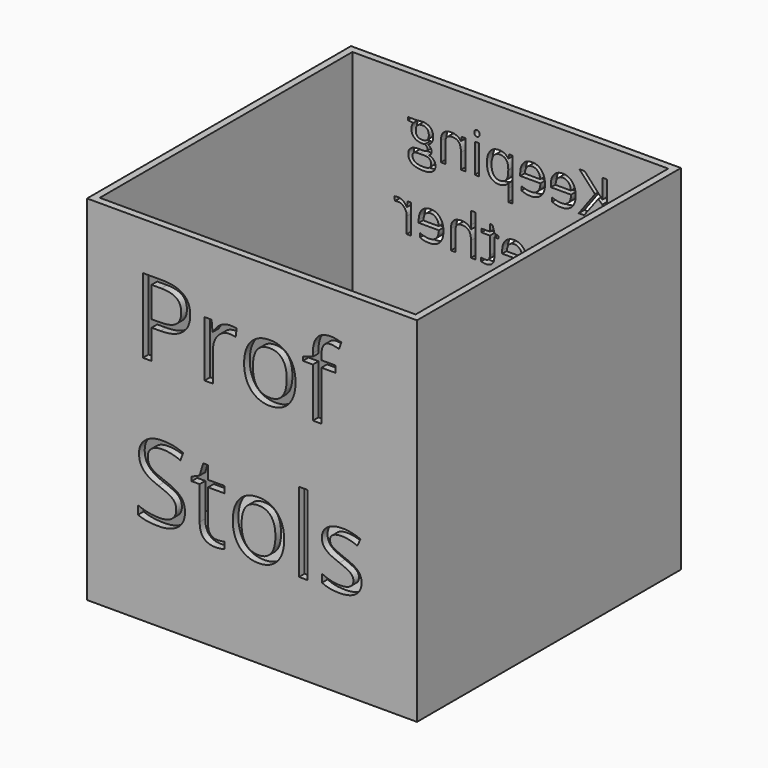
from build123d import *

# Parameters (mm, degrees)
F0_W         = 70
F0_H         = 70
F1_DEPTH     = 75
F2_W         = 67
F2_H         = 67
F3_DEPTH     = 70
F4_TEXT_SIZE = 22.1744854826
F5_DEPTH     = 5
F6_TEXT_SIZE = 11.5942028986
F7_DEPTH     = 5


# Not quite as in the source:
# - Text() gives the source's letters only with a copy of the font that has no kerning and outlines rounded to 1/6400 em; it was checked with that copy


with BuildPart() as f1:
    # F0 (on Top) → F1 (new body)
    with BuildSketch(Plane.XY):
        Rectangle(F0_W, F0_H)
    extrude(amount=F1_DEPTH)

    # F2 (on face) → F3 (cut)
    with BuildSketch(Plane.XY.offset(75)):
        Rectangle(F2_W, F2_H)
    extrude(amount=-F3_DEPTH, mode=Mode.SUBTRACT)

    # F4 (on face) → F5 (cut)
    with BuildSketch(Plane.XZ.offset(35)):
        with Locations((-25.3236840041, 49.0907604939)):
            Text('Prof', F4_TEXT_SIZE, font='Open Sans', text_align=(TextAlign.LEFT, TextAlign.BOTTOM))
        with Locations((-25.3236840041, 18.9334602375)):
            Text('Stols', F4_TEXT_SIZE, font='Open Sans', text_align=(TextAlign.LEFT, TextAlign.BOTTOM))
    extrude(amount=-F5_DEPTH, mode=Mode.SUBTRACT)

    # F6 (on face) → F7 (cut)
    with BuildSketch(Plane(origin=(0, 35, 0), x_dir=(-1, 0, 0), z_dir=(0, 1, 0))):
        with Locations((-21.6237345689, 60.4913517745)):
            Text('Keeping', F6_TEXT_SIZE, font='Open Sans', text_align=(TextAlign.LEFT, TextAlign.BOTTOM))
        with Locations((-21.6237345689, 44.7232358325)):
            Text('together', F6_TEXT_SIZE, font='Open Sans', text_align=(TextAlign.LEFT, TextAlign.BOTTOM))
        with Locations((-9.5730099312, 28.9551198904)):
            Text('the', F6_TEXT_SIZE, font='Open Sans', text_align=(TextAlign.LEFT, TextAlign.BOTTOM))
        with Locations((-24.6364157283, 13.1870039484)):
            Text('Coasters', F6_TEXT_SIZE, font='Open Sans', text_align=(TextAlign.LEFT, TextAlign.BOTTOM))
    extrude(amount=-F7_DEPTH, mode=Mode.SUBTRACT)


solid = f1.part
